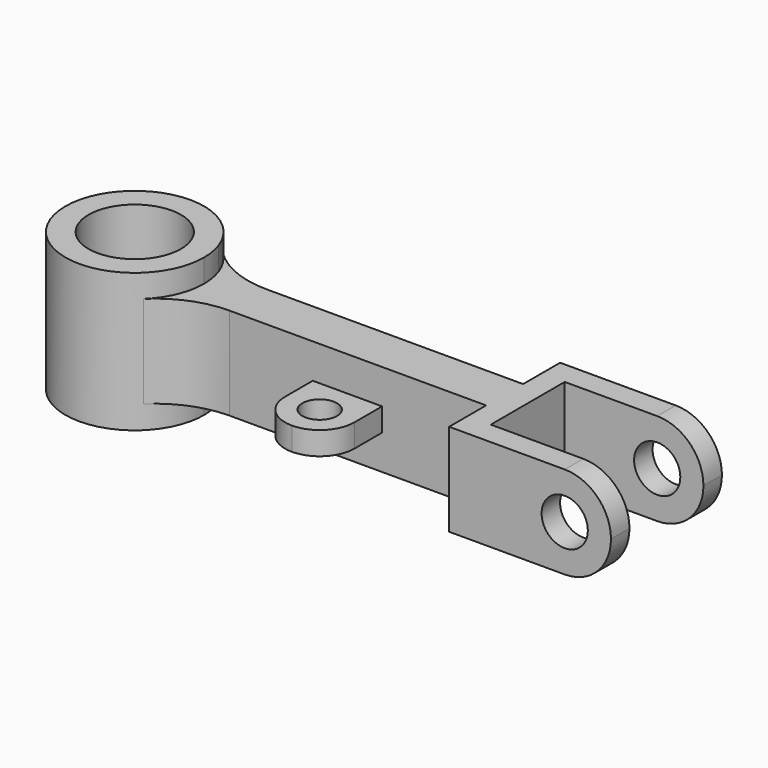
from build123d import *
from build123d import SkipClean  # not in build123d's __all__

# Parameters (mm, degrees)
F1_DEPTH    = 76.2
F3_DEPTH    = 12.7
F4_DEPTH    = 12.7
F5_T1_DEPTH = 50.8
F7_DEPTH    = 50.8
F8_R        = 25.39999
F9_R        = 12.7
F10_DEPTH   = 12.7
F13_DEPTH   = 38.1
F14_R       = 19.04999
F15_R       = 9.525
F16_DEPTH   = 12.7


# Not quite as in the source:
# - a fillet or chamfer that OpenCascade refuses, or shapes differently, is made with other operations: its cross-section is extruded or revolved along the edge and cut away or added
# - a fillet or chamfer is up to 0.001 mm smaller than in the source, because OpenCascade refuses the exact size


with BuildPart() as f1:
    # F0 (on Top) → F1 (new body)
    with BuildSketch(Plane.XY):
        with BuildLine():
            Line((-25.4, 0), (-38.1, 0))
            ThreePointArc((-38.1, 0), (-6.4427853895, -37.5513051228), (35.9210244843, -12.7))
            ThreePointArc((35.9210244843, -12.7), (37.5513051228, -6.4427853895), (38.1, 0))
            Line((38.1, 0), (25.4, 0))
            ThreePointArc((25.4, 0), (0, -25.4), (-25.4, 0))
        make_face()
        with BuildLine():
            ThreePointArc((38.1, 0), (37.5513051228, -6.4427853895), (35.9210244843, -12.7))
            Line((35.9210244843, -12.7), (203.2, -12.7))
            Line((203.2, -12.7), (203.2, 0))
            Line((203.2, 0), (38.1, 0))
        make_face()
    extrude(amount=F1_DEPTH)

    # F2 (on face) → F3 (cut)
    with BuildSketch(Plane.XY.offset(76.2)):
        with BuildLine():
            ThreePointArc((38.1, 0), (37.5513051228, -6.4427853895), (35.9210244843, -12.7))
            Line((35.9210244843, -12.7), (203.2, -12.7))
            Line((203.2, -12.7), (203.2, 0))
            Line((203.2, 0), (38.1, 0))
        make_face()
    extrude(amount=-F3_DEPTH, mode=Mode.SUBTRACT)

    # F0 (on Top) → F4 (cut)
    with BuildSketch(Plane.XY):
        with BuildLine():
            ThreePointArc((38.1, 0), (37.5513051228, -6.4427853895), (35.9210244843, -12.7))
            Line((35.9210244843, -12.7), (203.2, -12.7))
            Line((203.2, -12.7), (203.2, 0))
            Line((203.2, 0), (38.1, 0))
        make_face()
    extrude(amount=F4_DEPTH, mode=Mode.SUBTRACT)

    # F5: fillet of radius 50.8 on 1 edges, made by hand

    # F5_s2 → F5_t1 (join)
    with BuildSketch(Plane.XY.offset(12.7)):
        with BuildLine():
            ThreePointArc((62.2170394667, -12.7), (43.0164442378, -16.4683389316), (26.6644454857, -27.2142857143))
            ThreePointArc((26.6644454857, -27.2142857143), (32.1232219008, -20.4867912253), (35.9210244843, -12.7))
            Line((35.9210244843, -12.7), (62.2170394667, -12.7))
        make_face()
    extrude(amount=F5_T1_DEPTH)

    # F6 (on face) → F7 (join, through all)
    with BuildSketch(Plane.XY.offset(63.5)):
        Polygon((215.9, 0), (203.2, 0), (203.2, -12.7), (203.2, -38.1), (292.1, -38.1), (292.1, -25.4), (215.9, -25.4), align=None)
    extrude(amount=-F7_DEPTH)

    # F8 (radius 25.4 in the source; OpenCascade refuses exactly that, so slightly less here)
    f8_edges = [f1.edges().sort_by_distance(p)[0] for p in [
        (292.1, -31.75, 63.5),
        (292.1, -31.75, 12.7),
    ]]
    fillet(f8_edges, radius=F8_R)

    # F9 (on face) → F10 (cut, through all)
    with BuildSketch(Plane.XZ.offset(38.1)):
        with Locations((266.7, 38.1)):
            Circle(F9_R)
    extrude(amount=-F10_DEPTH, mode=Mode.SUBTRACT)

    # F11: F1 across plane


with BuildPart() as f1_1:
    add(f1.part, clean=False)
    with SkipClean():  # cleaning this boolean's faces spoils the solid; the shape is the same uncleaned
        add(f1.part.mirror(Plane.XZ), clean=False)

    # F12 (on face) → F13 (join)
    with BuildSketch(Plane.XZ.offset(12.7)):
        Polygon((146.05, 44.45), (127, 44.45), (107.95, 44.45), (107.95, 31.75), (127, 31.75), (146.05, 31.75), align=None)
    extrude(amount=F13_DEPTH)

    # F14 (radius 19.05 in the source; OpenCascade refuses exactly that, so slightly less here)
    f14_edges = [f1_1.edges().sort_by_distance(p)[0] for p in [
        (107.95, -50.8, 38.1),
        (146.05, -50.8, 38.1),
    ]]
    fillet(f14_edges, radius=F14_R)

    # F15 (on face) → F16 (cut, through all)
    with BuildSketch(Plane.XY.offset(44.45)):
        with Locations((127, -31.75)):
            Circle(F15_R)
    extrude(amount=-F16_DEPTH, mode=Mode.SUBTRACT)


solid = f1_1.part
